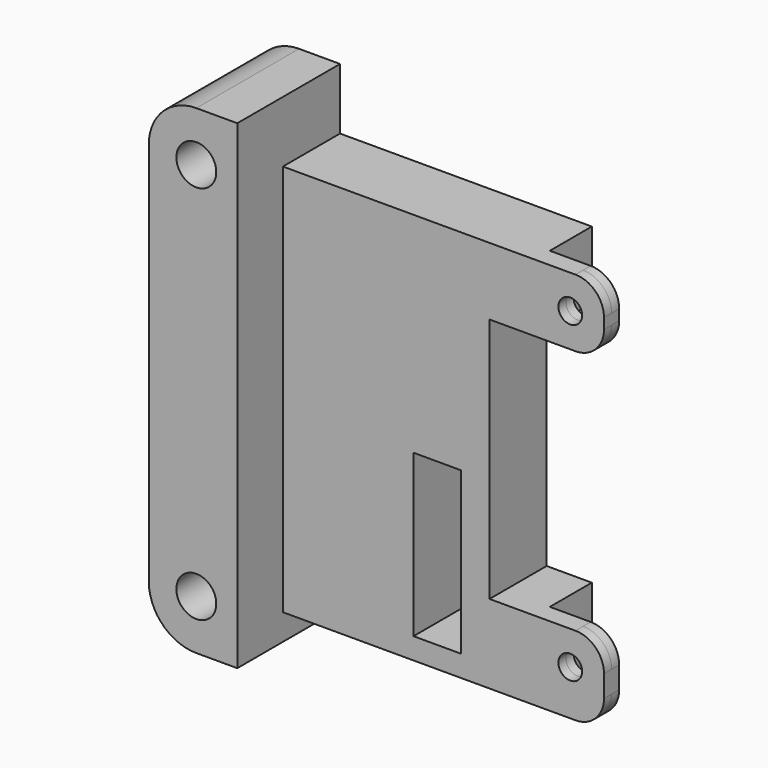
from build123d import *

# Parameters (mm, degrees)
F0_R          = 2.667
F0_R_2        = 1.5875
F0_W          = 6.35
F0_H          = 21.59
F1_DEPTH      = 1.27
F2_R          = 2.667
F3_DEPTH      = 8.2804
F3_DEPTH_BACK = 8.89
F4_W          = 2.396998
F4_H          = 10.541
F4_H_2        = 9.017
F5_DEPTH      = 25.4
F6_R          = 3.81
F7_W          = 6.35
F7_H          = 21.59
F8_DEPTH      = 8.2804
F9_R          = 1.5875
F10_DEPTH     = 1.27
F11_TEXT_SIZE = 23.6833103448
F12_DEPTH     = 1.524


# Not quite as in the source:
# - a feature names something its author has since deleted; it is built from what else it names
# - Text() gives the source's letters only with a copy of the font that has no kerning and outlines rounded to 1/6400 em; it was checked with that copy


with BuildPart() as f1:
    # F0 (on Front) → F1 (new body)
    with BuildSketch(Plane.XZ):
        with BuildLine():
            Line((-85.725, 0), (-136.525, 0))
            ThreePointArc((-136.525, 0), (-141.0151280605, -1.8598719395), (-142.875, -6.35))
            Line((-142.875, -6.35), (-142.875, -57.785))
            ThreePointArc((-142.875, -57.785), (-141.0151280605, -62.2751280605), (-136.525, -64.135))
            Line((-136.525, -64.135), (-85.725, -64.135))
            Line((-85.725, -64.135), (-85.725, 0))
        make_face()
        with Locations((-136.525, -57.4675)):
            Circle(F0_R, mode=Mode.SUBTRACT)
        with Locations((-92.630498, -54.61)):
            Circle(F0_R_2, mode=Mode.SUBTRACT)
        with Locations((-110.410625, -46.99)):
            Rectangle(F0_W, F0_H, mode=Mode.SUBTRACT)
        with Locations((-136.525, -6.6675)):
            Circle(F0_R, mode=Mode.SUBTRACT)
        with Locations((-92.630498, -12.7)):
            Circle(F0_R_2, mode=Mode.SUBTRACT)
    extrude(amount=F1_DEPTH)

    # F2 (on face) → F3 (join, two sides)
    with BuildSketch(Plane(origin=(0, 0, 0), x_dir=(-1, 0, 0), z_dir=(0, 1, 0))) as f3_sk:
        with BuildLine():
            Line((131.047998, 0), (131.047998, -64.135))
            Line((131.047998, -64.135), (136.525, -64.135))
            ThreePointArc((136.525, -64.135), (141.0151280605, -62.2751280605), (142.875, -57.785))
            Line((142.875, -57.785), (142.875, -6.35))
            ThreePointArc((142.875, -6.35), (141.0151280605, -1.8598719395), (136.525, 0))
            Line((136.525, 0), (131.047998, 0))
        make_face()
        with Locations((136.525, -57.4675)):
            Circle(F2_R, mode=Mode.SUBTRACT)
        with Locations((136.525, -6.6675)):
            Circle(F2_R, mode=Mode.SUBTRACT)
    extrude(amount=F3_DEPTH)
    extrude(f3_sk.sketch, amount=-F3_DEPTH_BACK)

    # F4 (on face) → F5 (cut)
    with BuildSketch(Plane(origin=(0, 0, 0), x_dir=(-1, 0, 0), z_dir=(0, 1, 0))):
        Polygon((88.121998, -17.2085), (85.725, -17.2085), (85.725, -50.1015), (88.121998, -50.1015), (103.425625, -50.1015), (103.425625, -17.2085), align=None)
        Polygon((131.047998, 0), (85.725, 0), (85.725, -8.1915), (88.121998, -8.1915), (131.047998, -8.1915), align=None)
        Polygon((131.047998, -64.135), (131.047998, -60.6425), (88.121998, -60.6425), (85.725, -60.6425), (85.725, -64.135), align=None)
        with Locations((86.923499, -55.372)):
            Rectangle(F4_W, F4_H)
        with Locations((86.923499, -12.7)):
            Rectangle(F4_W, F4_H_2)
    extrude(amount=-F5_DEPTH, mode=Mode.SUBTRACT)

    # F6
    f6_edges = [f1.edges().sort_by_distance(p)[0] for p in [
        (-88.121998, -0.635, -8.1915),
        (-88.121998, -0.635, -17.2085),
        (-88.121998, -0.635, -50.1015),
        (-88.121998, -0.635, -60.6425),
    ]]
    fillet(f6_edges, radius=F6_R)

    # F7 (on face) → F8 (join, through all)
    with BuildSketch(Plane(origin=(0, 0, 0), x_dir=(-1, 0, 0), z_dir=(0, 1, 0))):
        Polygon((131.047998, -60.6425), (131.047998, -8.1915), (97.392998, -8.1915), (97.392998, -17.2085), (103.425625, -17.2085), (103.425625, -50.1015), (97.392998, -50.1015), (97.392998, -60.6425), align=None)
        with Locations((110.410625, -46.99)):
            Rectangle(F7_W, F7_H, mode=Mode.SUBTRACT)
    extrude(amount=F8_DEPTH)

    # F9 (on face) → F10 (join)
    with BuildSketch(Plane(origin=(0, 0, 0), x_dir=(-1, 0, 0), z_dir=(0, 1, 0))):
        with BuildLine():
            Line((97.392998, -8.1915), (91.931998, -8.1915))
            ThreePointArc((91.931998, -8.1915), (89.2379211637, -9.3074231637), (88.121998, -12.0015))
            Line((88.121998, -12.0015), (88.121998, -13.3985))
            ThreePointArc((88.121998, -13.3985), (89.2379211637, -16.0925768363), (91.931998, -17.2085))
            Line((91.931998, -17.2085), (97.392998, -17.2085))
            Line((97.392998, -17.2085), (97.392998, -8.1915))
        make_face()
        with Locations((92.630498, -12.7)):
            Circle(F9_R, mode=Mode.SUBTRACT)
        with BuildLine():
            Line((97.392998, -50.1015), (91.931998, -50.1015))
            ThreePointArc((91.931998, -50.1015), (89.2379211637, -51.2174231637), (88.121998, -53.9115))
            Line((88.121998, -53.9115), (88.121998, -56.8325))
            ThreePointArc((88.121998, -56.8325), (89.2379211637, -59.5265768363), (91.931998, -60.6425))
            Line((91.931998, -60.6425), (97.392998, -60.6425))
            Line((97.392998, -60.6425), (97.392998, -50.1015))
        make_face()
        with Locations((92.630498, -54.61)):
            Circle(F9_R, mode=Mode.SUBTRACT)
    extrude(amount=F10_DEPTH)

    # F11 (on face) → F12 (cut)
    with BuildSketch(Plane(origin=(-142.875, 0, 0), x_dir=(0, -1, 0), z_dir=(-1, 0, 0))):
        with Locations((-8.2804, -40.9897888112)):
            Text('R', F11_TEXT_SIZE, font='Open Sans', font_style=FontStyle.BOLD, text_align=(TextAlign.LEFT, TextAlign.BOTTOM))
    extrude(amount=-F12_DEPTH, mode=Mode.SUBTRACT)


solid = f1.part
